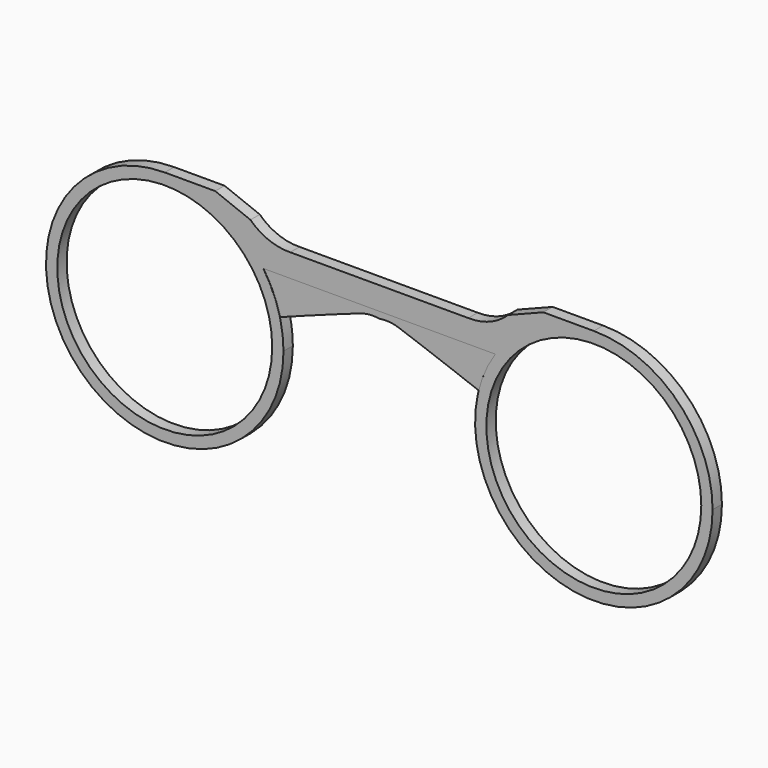
from build123d import *

# Parameters (mm, degrees)
F1_DEPTH = 1.5
F2_R     = 13.7922
F3_DEPTH = 25.4
F5_DEPTH = 25.4
F8_DEPTH = 1.4732


# Not quite as in the source:
# - a variable given as a bare number and used for a length is read in inches; the dataset says mm whatever the document's units were


with BuildPart() as f1:
    # F0 (on Front) → F1 (new body)
    with BuildSketch(Plane.XZ):
        with BuildLine():
            ThreePointArc((-27.5336, 15.24), (-38.3099073453, -10.7763073453), (-12.2936, 0))
            ThreePointArc((-12.2936, 0), (-12.9572083605, 4.4481914045), (-14.8902413086, 8.509))
            ThreePointArc((-14.8902413086, 8.509), (-20.3718809326, 13.4524116797), (-27.5336, 15.24))
        make_face()
        with BuildLine():
            ThreePointArc((-27.5336, 15.24), (-20.3718809326, 13.4524116797), (-14.8902413086, 8.509))
            Line((-14.8902413086, 8.509), (14.8902413086, 8.509))
            ThreePointArc((14.8902413086, 8.509), (20.3718809326, 13.4524116797), (27.5336, 15.24))
            Line((27.5336, 15.24), (-27.5336, 15.24))
        make_face()
        with BuildLine():
            ThreePointArc((27.5336, 15.24), (20.3718809326, 13.4524116797), (14.8902413086, 8.509))
            ThreePointArc((14.8902413086, 8.509), (23.0854085955, -14.5763916395), (42.7736, 0))
            ThreePointArc((42.7736, 0), (38.3099073453, 10.7763073453), (27.5336, 15.24))
        make_face()
    extrude(amount=F1_DEPTH)

    # F2 (on face) → F3 (cut)
    with BuildSketch(Plane.XZ.offset(1.5)):
        with Locations((-27.5336, 0)):
            Circle(F2_R)
        with Locations((27.5336, 0)):
            Circle(F2_R)
        with BuildLine():
            Line((0, 40.3644442558), (-21.547392987, 18.4778384864))
            Line((-21.547392987, 18.4778384864), (-16.5919354635, 13.522380963))
            ThreePointArc((-16.5919354635, 13.522380963), (-14.2228731292, 11.9602304674), (-11.43, 11.4576071501))
            Line((-11.43, 11.4576071501), (0, 11.4576071501))
            Line((0, 11.4576071501), (0, 40.3644442558))
        make_face()
        with BuildLine():
            Line((21.547392987, 18.4778384864), (0, 40.3644442558))
            Line((0, 40.3644442558), (0, 11.4576071501))
            Line((0, 11.4576071501), (11.43, 11.4576071501))
            ThreePointArc((11.43, 11.4576071501), (14.2228731292, 11.9602304674), (16.5919354635, 13.522380963))
            Line((16.5919354635, 13.522380963), (21.547392987, 18.4778384864))
        make_face()
    extrude(amount=-F3_DEPTH, mode=Mode.SUBTRACT)

    # F4 (on face) → F5 (cut)
    with BuildSketch(Plane.XZ.offset(1.5)):
        Polygon((-9.2328525533, 17.0485330061), (-24.6466696262, 16.6515540332), (-11.43, 11.4576071501), align=None)
        Polygon((11.43, 11.4576071501), (24.6466696262, 16.6515540332), (9.2328525533, 17.0485330061), align=None)
    extrude(amount=-F5_DEPTH, mode=Mode.SUBTRACT)

    # F7 (on Front) → F8 (join)
    with BuildSketch(Plane.XZ):
        with BuildLine():
            ThreePointArc((-17.6120530814, 10.0212339312), (-15.0131826274, 7.0473877292), (-13.4240113708, 3.4318070584))
            ThreePointArc((-13.4240113708, 3.4318070584), (-7.9783410744, 5.4701683575), (-2.5081751928, 7.4418496173))
            ThreePointArc((-2.5081751928, 7.4418496173), (-1.2673351307, 7.7068584172), (0, 7.6454142109))
            ThreePointArc((0, 7.6454142109), (1.2673351307, 7.7068584172), (2.5081751928, 7.4418496173))
            ThreePointArc((2.5081751928, 7.4418496173), (7.9783410744, 5.4701683575), (13.4240113708, 3.4318070584))
            ThreePointArc((13.4240113708, 3.4318070584), (15.0131826274, 7.0473877292), (17.6120530814, 10.0212339312))
            Line((17.6120530814, 10.0212339312), (-17.6120530814, 10.0212339312))
        make_face()
    extrude(amount=F8_DEPTH)


solid = f1.part
